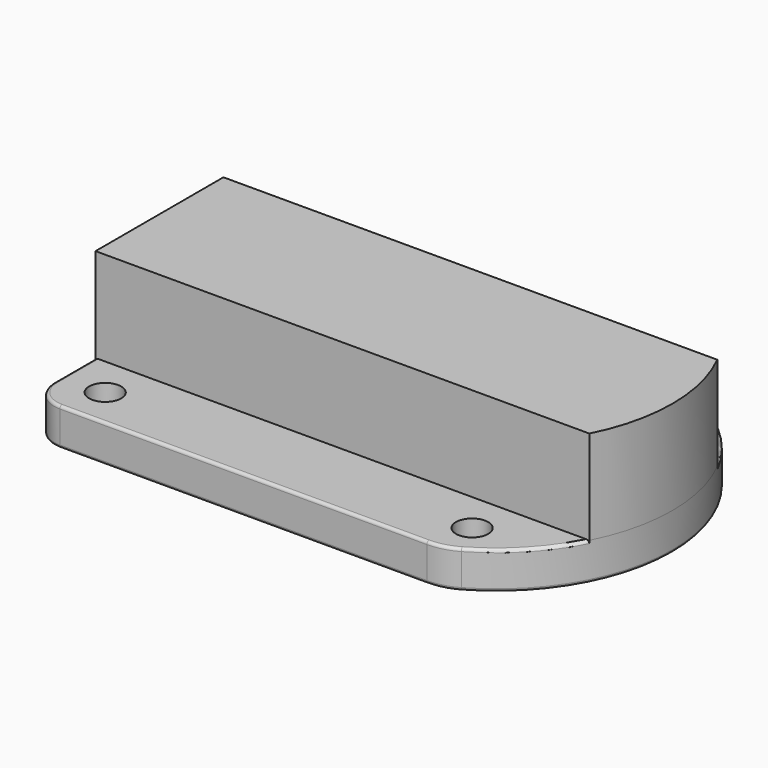
from build123d import *

# Parameters (mm, degrees)
F0_R         = 2.8
F1_DEPTH     = 6.5
F3_DEPTH     = 16.35
F4_T1_DEPTH  = 63.8184719387
F4_T3_DEPTH  = 45.8
F4_T5_DEPTH  = 9
F4_T7_DEPTH  = 9
F4_T10_ANGLE = 90
F4_T12_ANGLE = 120.4504110916
F4_T14_ANGLE = 90
F4_T16_ANGLE = 90
F4_T18_ANGLE = 29.7747944542
F4_T20_ANGLE = 29.7747944542
F4_T22_ANGLE = 29.7747944542
F4_T26_ANGLE = 35.5690080159
F4_T29_ANGLE = 90
F4_T33_ANGLE = 35.5690080159
F4_T36_ANGLE = 29.7747944542
F5_SIZE      = 1.56


# Not quite as in the source:
# - a fillet or chamfer that OpenCascade refuses, or shapes differently, is made with other operations: its cross-section is extruded or revolved along the edge and cut away or added


with BuildPart() as f1:
    # F0 (on Top) → F1 (new body)
    with BuildSketch(Plane.XY):
        with BuildLine():
            Line((-38.8770699501, 16.9000072956), (-38.8770699501, -28.8999927044))
            ThreePointArc((-38.8770699501, -28.8999927044), (-37.412603856, -32.4355266103), (-33.8770699501, -33.8999927044))
            Line((-33.8770699501, -33.8999927044), (29.9414019886, -33.8999927044))
            ThreePointArc((29.9414019886, -33.8999927044), (32.5106042183, -33.5643188528), (34.9073236464, -32.579832685))
            ThreePointArc((34.9073236464, -32.579832685), (50.3229300499, -5.9999927044), (34.9073236464, 20.5798472762))
            ThreePointArc((34.9073236464, 20.5798472762), (32.5106042183, 21.564333444), (29.9414019886, 21.9000072956))
            Line((29.9414019886, 21.9000072956), (-33.8770699501, 21.9000072956))
            ThreePointArc((-33.8770699501, 21.9000072956), (-37.412603856, 20.4355412015), (-38.8770699501, 16.9000072956))
        make_face()
        with Locations((-31.5170697868, -26.9999932498)):
            Circle(F0_R, mode=Mode.SUBTRACT)
        with Locations((32.2829300499, -26.9999927044)):
            Circle(F0_R, mode=Mode.SUBTRACT)
        with Locations((-31.5170697868, 15.0000071153)):
            Circle(F0_R, mode=Mode.SUBTRACT)
        with Locations((32.2829300499, 15.0000072956)):
            Circle(F0_R, mode=Mode.SUBTRACT)
    extrude(amount=F1_DEPTH)

    # F2 (on face) → F3 (join)
    with BuildSketch(Plane.XY.offset(6.5)):
        with BuildLine():
            Line((-38.8770699501, 7.9000072956), (-38.8770699501, -5.9999927044))
            Line((-38.8770699501, -5.9999927044), (-38.8770699501, -19.8999927044))
            Line((-38.8770699501, -19.8999927044), (46.9864613892, -19.8999927044))
            ThreePointArc((46.9864613892, -19.8999927044), (50.3229300499, -5.9999927044), (46.9864613892, 7.9000072956))
            Line((46.9864613892, 7.9000072956), (-38.8770699501, 7.9000072956))
        make_face()
    extrude(amount=F3_DEPTH)

    # F4: fillet of radius 0.5 on 18 edges, made by hand

    # F4_s2 → F4_t1 (cut)
    with BuildSketch(Plane.YZ.offset(-33.8770699501)):
        with BuildLine():
            ThreePointArc((21.9000072956, 0.5), (21.7535606862, 0.1464466094), (21.4000072956, 0))
            Line((21.4000072956, 0), (21.9000072956, 0))
            Line((21.9000072956, 0), (21.9000072956, 0.5))
        make_face()
        with BuildLine():
            ThreePointArc((21.9000072956, 6), (21.7535606862, 6.3535533906), (21.4000072956, 6.5))
            Line((21.4000072956, 6.5), (21.9000072956, 6.5))
            Line((21.9000072956, 6.5), (21.9000072956, 6))
        make_face()
        with BuildLine():
            ThreePointArc((-33.3999927044, 6.5), (-33.753546095, 6.3535533906), (-33.8999927044, 6))
            Line((-33.8999927044, 6), (-33.8999927044, 6.5))
            Line((-33.8999927044, 6.5), (-33.3999927044, 6.5))
        make_face()
        with BuildLine():
            ThreePointArc((-33.3999927044, 0), (-33.753546095, 0.1464466094), (-33.8999927044, 0.5))
            Line((-33.8999927044, 0.5), (-33.8999927044, 0))
            Line((-33.8999927044, 0), (-33.3999927044, 0))
        make_face()
    extrude(amount=F4_T1_DEPTH, mode=Mode.SUBTRACT)

    # F4_s4 → F4_t3 (cut)
    with BuildSketch(Plane.XZ.offset(-16.9000072956)):
        with BuildLine():
            ThreePointArc((-38.8770699501, 0.5), (-38.7306233407, 0.1464466094), (-38.3770699501, 0))
            Line((-38.3770699501, 0), (-38.8770699501, 0))
            Line((-38.8770699501, 0), (-38.8770699501, 0.5))
        make_face()
    extrude(amount=F4_T3_DEPTH, mode=Mode.SUBTRACT)

    # F4_s6 → F4_t5 (cut)
    with BuildSketch(Plane.XZ.offset(-16.9000072956)):
        with BuildLine():
            ThreePointArc((-38.8770699501, 6), (-38.7306233407, 6.3535533906), (-38.3770699501, 6.5))
            Line((-38.3770699501, 6.5), (-38.8770699501, 6.5))
            Line((-38.8770699501, 6.5), (-38.8770699501, 6))
        make_face()
    extrude(amount=F4_T5_DEPTH, mode=Mode.SUBTRACT)

    # F4_s8 → F4_t7 (cut)
    with BuildSketch(Plane.XZ.offset(19.8999927044)):
        with BuildLine():
            ThreePointArc((-38.8770699501, 6), (-38.7306233407, 6.3535533906), (-38.3770699501, 6.5))
            Line((-38.3770699501, 6.5), (-38.8770699501, 6.5))
            Line((-38.8770699501, 6.5), (-38.8770699501, 6))
        make_face()
    extrude(amount=F4_T7_DEPTH, mode=Mode.SUBTRACT)

    # F4_s9 → F4_t10 (revolve, cut)
    with BuildSketch(Plane.YZ.offset(-33.8770699501)):
        with BuildLine():
            ThreePointArc((21.9000072956, 0.5), (21.7535606862, 0.1464466094), (21.4000072956, 0))
            Line((21.4000072956, 0), (21.9000072956, 0))
            Line((21.9000072956, 0), (21.9000072956, 0.5))
        make_face()
    revolve(axis=Axis((-33.8770699501, 16.9000072956, 0), (0, 0, 1)), revolution_arc=F4_T10_ANGLE, mode=Mode.SUBTRACT)

    # F4_s11 → F4_t12 (revolve, cut)
    with BuildSketch(Plane(origin=(12.2560283734, 7.0119353437, 0), x_dir=(0, 0, 1), z_dir=(-0.8679839981, -0.4965921658, 0))):
        with BuildLine():
            ThreePointArc((0, -45.1134768811), (0.1464466094, -45.4670302717), (0.5, -45.6134768811))
            Line((0.5, -45.6134768811), (0, -45.6134768811))
            Line((0, -45.6134768811), (0, -45.1134768811))
        make_face()
    revolve(axis=Axis((19.7004300499, -5.9999927044, 0), (0, 0, 1)), revolution_arc=F4_T12_ANGLE, mode=Mode.SUBTRACT)

    # F4_s13 → F4_t14 (revolve, cut)
    with BuildSketch(Plane.YZ.offset(-33.8770699501)):
        with BuildLine():
            ThreePointArc((21.9000072956, 6), (21.7535606862, 6.3535533906), (21.4000072956, 6.5))
            Line((21.4000072956, 6.5), (21.9000072956, 6.5))
            Line((21.9000072956, 6.5), (21.9000072956, 6))
        make_face()
    revolve(axis=Axis((-33.8770699501, 16.9000072956, 6.5), (0, 0, 1)), revolution_arc=F4_T14_ANGLE, mode=Mode.SUBTRACT)

    # F4_s15 → F4_t16 (revolve, cut)
    with BuildSketch(Plane.XZ.offset(28.8999927044)):
        with BuildLine():
            ThreePointArc((-38.3770699501, 0), (-38.7306233407, 0.1464466094), (-38.8770699501, 0.5))
            Line((-38.8770699501, 0.5), (-38.8770699501, 0))
            Line((-38.8770699501, 0), (-38.3770699501, 0))
        make_face()
    revolve(axis=Axis((-33.8770699501, -28.8999927044, 0), (0, 0, 1)), revolution_arc=F4_T16_ANGLE, mode=Mode.SUBTRACT)

    # F4_s17 → F4_t18 (revolve, cut)
    with BuildSketch(Plane.YZ.offset(29.9414019886)):
        with BuildLine():
            ThreePointArc((-33.3999927044, 0), (-33.753546095, 0.1464466094), (-33.8999927044, 0.5))
            Line((-33.8999927044, 0.5), (-33.8999927044, 0))
            Line((-33.8999927044, 0), (-33.3999927044, 0))
        make_face()
    revolve(axis=Axis((29.9414019886, -23.8999927044, 0), (0, 0, 1)), revolution_arc=F4_T18_ANGLE, mode=Mode.SUBTRACT)

    # F4_s19 → F4_t20 (revolve, cut)
    with BuildSketch(Plane(origin=(17.4284307256, -9.9711770948, 0), x_dir=(0, 0, 1), z_dir=(0.8679839981, -0.4965921658, 0))):
        with BuildLine():
            ThreePointArc((0, -34.6976815693), (0.1464466094, -35.0512349599), (0.5, -35.1976815693))
            Line((0.5, -35.1976815693), (0, -35.1976815693))
            Line((0, -35.1976815693), (0, -34.6976815693))
        make_face()
    revolve(axis=Axis((29.9414019886, 11.9000072956, 0), (0, 0, 1)), revolution_arc=F4_T20_ANGLE, mode=Mode.SUBTRACT)

    # F4_s21 → F4_t22 (revolve, cut)
    with BuildSketch(Plane(origin=(17.4284307256, -9.9711770948, 0), x_dir=(0, 0, 1), z_dir=(0.8679839981, -0.4965921658, 0))):
        with BuildLine():
            ThreePointArc((6.5, -34.6976815693), (6.3535533906, -35.0512349599), (6, -35.1976815693))
            Line((6, -35.1976815693), (6.5, -35.1976815693))
            Line((6.5, -35.1976815693), (6.5, -34.6976815693))
        make_face()
    revolve(axis=Axis((29.9414019886, 11.9000072956, 6.5), (0, 0, 1)), revolution_arc=F4_T22_ANGLE, mode=Mode.SUBTRACT)


with BuildPart() as f4_tool24:
    # F4_s25 → F4_t26 (revolve)
    with BuildSketch(Plane(origin=(5.7033446243, -12.4249727464, 0), x_dir=(0, 0, 1), z_dir=(0.4171723997, -0.9088273703, 0))):
        with BuildLine():
            ThreePointArc((6.5, -45.5237586807), (6.3535533906, -45.8773120713), (6, -46.0237586807))
            Line((6, -46.0237586807), (6.5, -46.0237586807))
            Line((6.5, -46.0237586807), (6.5, -45.5237586807))
        make_face()
    revolve(axis=Axis((19.7004300499, -5.9999927044, 6.5), (0, 0, 1)), revolution_arc=F4_T26_ANGLE)

    split(bisect_by=Plane.XZ.offset(-7.9000072956), keep=Keep.BOTTOM)


with BuildPart() as f1_1:
    add(f1.part)

    # F4_t23: cut F4_tool24
    add(f4_tool24.part, mode=Mode.SUBTRACT)

    # F4_s28 → F4_t29 (revolve, cut)
    with BuildSketch(Plane.XZ.offset(28.8999927044)):
        with BuildLine():
            ThreePointArc((-38.8770699501, 6), (-38.7306233407, 6.3535533906), (-38.3770699501, 6.5))
            Line((-38.3770699501, 6.5), (-38.8770699501, 6.5))
            Line((-38.8770699501, 6.5), (-38.8770699501, 6))
        make_face()
    revolve(axis=Axis((-33.8770699501, -28.8999927044, 6.5), (0, 0, 1)), revolution_arc=F4_T29_ANGLE, mode=Mode.SUBTRACT)


with BuildPart() as f4_tool31:
    # F4_s32 → F4_t33 (revolve)
    with BuildSketch(Plane(origin=(12.2560283734, 7.0119353437, 0), x_dir=(0, 0, 1), z_dir=(-0.8679839981, -0.4965921658, 0))):
        with BuildLine():
            ThreePointArc((6.5, -45.1134768811), (6.3535533906, -45.4670302717), (6, -45.6134768811))
            Line((6, -45.6134768811), (6.5, -45.6134768811))
            Line((6.5, -45.6134768811), (6.5, -45.1134768811))
        make_face()
    revolve(axis=Axis((19.7004300499, -5.9999927044, 6.5), (0, 0, 1)), revolution_arc=F4_T33_ANGLE)

    split(bisect_by=Plane.XZ.offset(19.8999927044), keep=Keep.TOP)


with BuildPart() as f1_2:
    add(f1_1.part)

    # F4_t30: cut F4_tool31
    add(f4_tool31.part, mode=Mode.SUBTRACT)

    # F4_s35 → F4_t36 (revolve, cut)
    with BuildSketch(Plane.YZ.offset(29.9414019886)):
        with BuildLine():
            ThreePointArc((-33.3999927044, 6.5), (-33.753546095, 6.3535533906), (-33.8999927044, 6))
            Line((-33.8999927044, 6), (-33.8999927044, 6.5))
            Line((-33.8999927044, 6.5), (-33.3999927044, 6.5))
        make_face()
    revolve(axis=Axis((29.9414019886, -23.8999927044, 6.5), (0, 0, 1)), revolution_arc=F4_T36_ANGLE, mode=Mode.SUBTRACT)

    # F5
    f5_edges = [f1_2.edges().sort_by_distance(p)[0] for p in [
        (-34.31707, 15.000007, 0),
        (-34.31707, -26.999993, 0),
        (29.48293, -26.999993, 0),
        (29.48293, 15.000007, 0),
    ]]
    chamfer(f5_edges, length=F5_SIZE)


solid = f1_2.part
